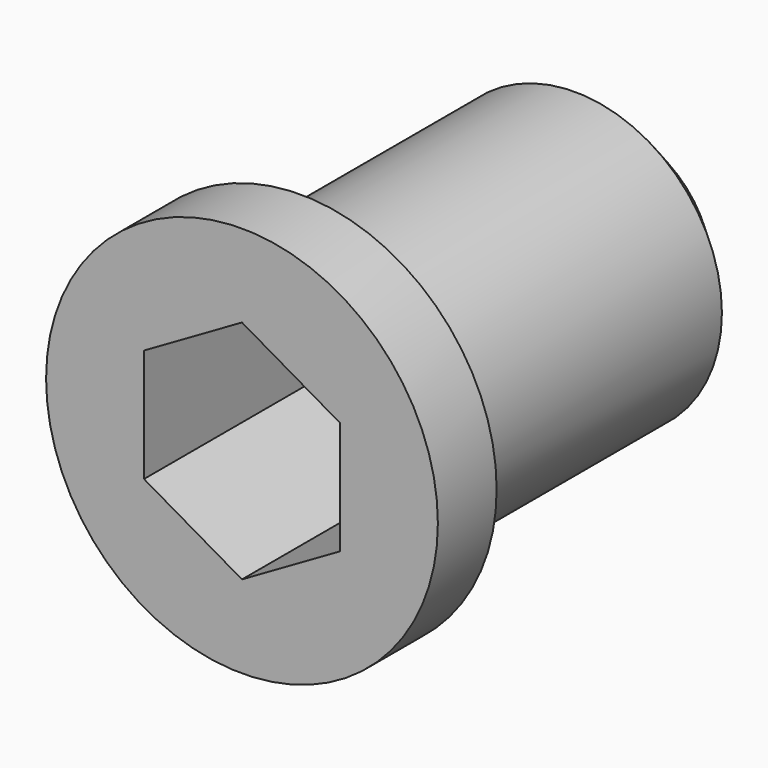
from build123d import *

# Parameters (mm, degrees)
F0_R     = 3
F1_DEPTH = 8
F3_DEPTH = 3
F4_R     = 2
F5_DEPTH = 25
F6_SIZE  = 0.99999
F7_R     = 4
F8_DEPTH = 1.5


# Not quite as in the source:
# - a fillet or chamfer is up to 0.001 mm smaller than in the source, because OpenCascade refuses the exact size


with BuildPart() as f1:
    # F0 (on Front) → F1 (new body)
    with BuildSketch(Plane.XZ):
        Circle(F0_R)
    extrude(amount=F1_DEPTH)

    # F2 (on face) → F3 (cut)
    with BuildSketch(Plane.XZ.offset(8)):
        Polygon((2, 1.1547005384), (0, 2.3094010768), (-2, 1.1547005384), (-2, -1.1547005384), (0, -2.3094010768), (2, -1.1547005384), align=None)
    extrude(amount=-F3_DEPTH, mode=Mode.SUBTRACT)

    # F4 (on face) → F5 (cut)
    with BuildSketch(Plane.XZ.offset(5)):
        Circle(F4_R)
    extrude(amount=-F5_DEPTH, mode=Mode.SUBTRACT)

    # F6 (size 1 in the source; OpenCascade refuses exactly that, so slightly less here)
    f6_edges = [f1.edges().sort_by_distance(p)[0] for p in [
        (-3, 0, 0),
    ]]
    chamfer(f6_edges, length=F6_SIZE)

    # F7 (on face) → F8 (join)
    with BuildSketch(Plane.XZ.offset(8)):
        Circle(F7_R)
        Polygon((2, 1.1547005384), (2, -1.1547005384), (0, -2.3094010768), (-2, -1.1547005384), (-2, 1.1547005384), (0, 2.3094010768), align=None, mode=Mode.SUBTRACT)
    extrude(amount=F8_DEPTH)


solid = f1.part
